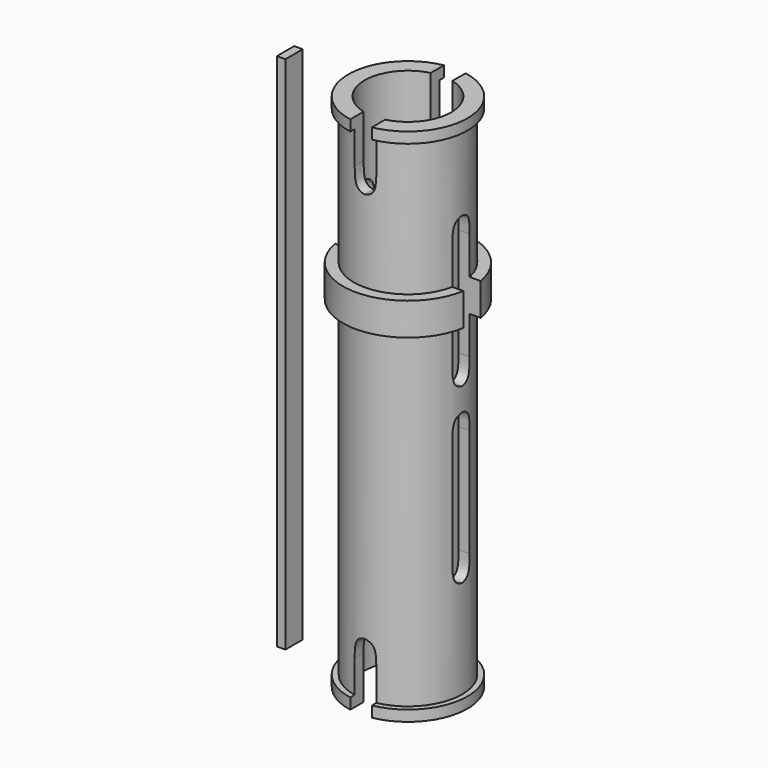
from build123d import *

# Parameters (mm, degrees)
F0_R           = 3
F1_DEPTH       = 24
F2_R           = 3
F2_R_2         = 2.5
F3_DEPTH       = 6.75
F4_R           = 2.75
F5_DEPTH       = 0.5
F6_R           = 3
F6_R_2         = 2.5
F7_DEPTH       = 6.75
F8_R           = 2.75
F9_DEPTH       = 0.5
F10_R          = 2
F11_DEPTH      = 25
F13_DEPTH      = 3
F15_DEPTH      = 3
F16_DEPTH      = 9
F17_T4_DEPTH   = 5.5129980697
F17_S5_R       = 2.5
F17_T6_DEPTH   = 4
F17_S7_R       = 2
F17_T8_DEPTH   = 4
F17_T12_DEPTH  = 5.5129980697
F17_S13_R      = 2.5
F17_T14_DEPTH  = 4
F17_S15_R      = 2
F17_T16_DEPTH  = 4
F17_T20_DEPTH  = 5.5129980697
F17_S21_R      = 2.5
F17_T22_DEPTH  = 4
F17_S23_R      = 2
F17_T24_DEPTH  = 4
F17_T28_DEPTH  = 5.5129980697
F17_S29_R      = 2.5
F17_T30_DEPTH  = 4
F17_S31_R      = 2
F17_T32_DEPTH  = 4
F17_T36_DEPTH  = 5.5129980697
F17_S37_R      = 2
F17_T38_DEPTH  = 4
F17_S39_R      = 2.5
F17_T40_DEPTH  = 4
F17_T44_DEPTH  = 5.5129980697
F17_S45_R      = 2
F17_T46_DEPTH  = 4
F17_S47_R      = 2.5
F17_T48_DEPTH  = 4
F17_T52_DEPTH  = 5.5129980697
F17_S53_R      = 2
F17_T54_DEPTH  = 4
F17_S55_R      = 2.5
F17_T56_DEPTH  = 4
F17_T60_DEPTH  = 5.5129980697
F17_S61_R      = 2
F17_T62_DEPTH  = 4
F17_S63_R      = 2.5
F17_T64_DEPTH  = 4
F19_DEPTH      = 24
F20_W          = 1
F20_H          = 7
F21_DEPTH      = 25
F22_T4_DEPTH   = 5.5129980697
F22_S5_R       = 2
F22_T6_DEPTH   = 4
F22_S7_R       = 2.5
F22_T8_DEPTH   = 4
F22_T12_DEPTH  = 5.5129980697
F22_S13_R      = 2
F22_T14_DEPTH  = 4
F22_S15_R      = 2.5
F22_T16_DEPTH  = 4
F22_T20_DEPTH  = 5.5129980697
F22_S21_R      = 2
F22_T22_DEPTH  = 4
F22_S23_R      = 2.5
F22_T24_DEPTH  = 4
F22_T28_DEPTH  = 5.5129980697
F22_S29_R      = 2
F22_T30_DEPTH  = 4
F22_S31_R      = 2.5
F22_T32_DEPTH  = 4
F22_T36_DEPTH  = 5.5129980697
F22_S37_R      = 2
F22_T38_DEPTH  = 4
F22_S39_R      = 2.5
F22_T40_DEPTH  = 4
F22_T44_DEPTH  = 5.5129980697
F22_S45_R      = 2
F22_T46_DEPTH  = 4
F22_S47_R      = 2.5
F22_T48_DEPTH  = 4
F22_T52_DEPTH  = 5.5129980697
F22_S53_R      = 2
F22_T54_DEPTH  = 4
F22_S55_R      = 2.5
F22_T56_DEPTH  = 4
F22_T60_DEPTH  = 5.5129980697
F22_S61_R      = 2
F22_T62_DEPTH  = 4
F22_S63_R      = 2.5
F22_T64_DEPTH  = 4
F22_T68_DEPTH  = 5.5129980697
F22_S69_R      = 2
F22_T70_DEPTH  = 4
F22_S71_R      = 2.5
F22_T72_DEPTH  = 4
F22_T76_DEPTH  = 5.5129980697
F22_S77_R      = 2
F22_T78_DEPTH  = 4
F22_S79_R      = 2.5
F22_T80_DEPTH  = 4
F22_T84_DEPTH  = 5.5129980697
F22_S85_R      = 2
F22_T86_DEPTH  = 4
F22_S87_R      = 2.5
F22_T88_DEPTH  = 4
F22_T92_DEPTH  = 5.5129980697
F22_S93_R      = 2.5
F22_T94_DEPTH  = 4
F22_S95_R      = 2
F22_T96_DEPTH  = 4
F22_T100_DEPTH = 5.5129980697
F22_S101_R     = 2
F22_T102_DEPTH = 4
F22_S103_R     = 2.5
F22_T104_DEPTH = 4
F22_T108_DEPTH = 5.5129980697
F22_S109_R     = 2.5
F22_T110_DEPTH = 4
F22_S111_R     = 2
F22_T112_DEPTH = 4
F22_T116_DEPTH = 5.5129980697
F22_S117_R     = 2
F22_T118_DEPTH = 4
F22_S119_R     = 2.5
F22_T120_DEPTH = 4
F22_T124_DEPTH = 5.5129980697
F22_S125_R     = 2
F22_T126_DEPTH = 4
F22_S127_R     = 2.5
F22_T128_DEPTH = 4


# Not quite as in the source:
# - a fillet or chamfer that OpenCascade refuses, or shapes differently, is made with other operations: its cross-section is extruded or revolved along the edge and cut away or added


with BuildPart() as f1:
    # F0 (on Top) → F1 (new body)
    with BuildSketch(Plane.XY):
        with Locations((-5.9236139059, -29.9984049052)):
            Circle(F0_R)
    extrude(amount=F1_DEPTH)

    # F2 (on face) → F3 (cut)
    with BuildSketch(Plane.XY.offset(24)):
        with Locations((-5.9236139059, -29.9984049052)):
            Circle(F2_R)
        with Locations((-5.9236139059, -29.9984049052)):
            Circle(F2_R_2, mode=Mode.SUBTRACT)
    extrude(amount=-F3_DEPTH, mode=Mode.SUBTRACT)

    # F4 (on face) → F5 (join)
    with BuildSketch(Plane.XY.offset(24)):
        with Locations((-5.9236139059, -29.9984049052)):
            Circle(F4_R)
    extrude(amount=-F5_DEPTH)

    # F6 (on face) → F7 (cut)
    with BuildSketch(Plane(origin=(0, 0, 0), x_dir=(1, 0, 0), z_dir=(0, 0, -1))):
        with Locations((-5.9236139059, 29.9984049052)):
            Circle(F6_R)
        with Locations((-5.9236139059, 29.9984049052)):
            Circle(F6_R_2, mode=Mode.SUBTRACT)
    extrude(amount=-F7_DEPTH, mode=Mode.SUBTRACT)

    # F8 (on face) → F9 (join)
    with BuildSketch(Plane(origin=(0, 0, 0), x_dir=(1, 0, 0), z_dir=(0, 0, -1))):
        with Locations((-5.9236139059, 29.9984049052)):
            Circle(F8_R)
    extrude(amount=-F9_DEPTH)

    # F10 (on face) → F11 (cut)
    with BuildSketch(Plane(origin=(0, 0, 0), x_dir=(1, 0, 0), z_dir=(0, 0, -1))):
        with Locations((-5.9236139059, 29.9984049052)):
            Circle(F10_R)
    extrude(amount=-F11_DEPTH, mode=Mode.SUBTRACT)

    # F12 (on face) → F13 (cut)
    with BuildSketch(Plane.XY.offset(24)):
        with BuildLine():
            ThreePointArc((-6.4236139059, -32.7025683618), (-5.9236139059, -32.7484049052), (-5.4236139059, -32.7025683618))
            Line((-5.4236139059, -32.7025683618), (-5.4236139059, -31.9348965783))
            ThreePointArc((-5.4236139059, -31.9348965783), (-5.9236139059, -31.9984049052), (-6.4236139059, -31.9348965783))
            Line((-6.4236139059, -31.9348965783), (-6.4236139059, -32.7025683618))
        make_face()
        with BuildLine():
            ThreePointArc((-5.4236139059, -27.2942414486), (-5.9236139059, -27.2484049052), (-6.4236139059, -27.2942414486))
            Line((-6.4236139059, -27.2942414486), (-6.4236139059, -28.0619132321))
            ThreePointArc((-6.4236139059, -28.0619132321), (-5.9236139059, -27.9984049052), (-5.4236139059, -28.0619132321))
            Line((-5.4236139059, -28.0619132321), (-5.4236139059, -27.2942414486))
        make_face()
    extrude(amount=-F13_DEPTH, mode=Mode.SUBTRACT)

    # F14 (on face) → F15 (cut)
    with BuildSketch(Plane(origin=(0, 0, 0), x_dir=(1, 0, 0), z_dir=(0, 0, -1))):
        Polygon((-5.4236139059, 33.0966450274), (-5.9236139059, 33.0966450274), (-6.4236139059, 33.0966450274), (-6.4236139059, 26.7786514014), (-5.4236139059, 26.7786514014), align=None)
    extrude(amount=-F15_DEPTH, mode=Mode.SUBTRACT)

    # F16 (cut): a face of the model
    f16_faces = [f1.faces().sort_by_distance(p)[0] for p in [
        (-8.8387610922, -29.9984049052, 6.75),
    ]]
    extrude(f16_faces, amount=-F16_DEPTH, mode=Mode.SUBTRACT)

    # F17: fillet of radius 1 on 8 edges, made by hand


with BuildPart() as f17_tool2:
    # F17_s3 → F17_t4 (new body)
    with BuildSketch(Plane.XZ.offset(29.4348965783)):
        with BuildLine():
            add(Edge.make_bspline(
                [(-5.4236139059, 21), (-6.4236139059, 21), (-6.4236139059, 22)],
                knots=[0, 0, 0, 1, 1, 1], degree=2, weights=[1, 1.8571428571, 1]))
            Line((-6.4236139059, 22), (-6.4236139059, 21))
            Line((-6.4236139059, 21), (-5.4236139059, 21))
        make_face()
    extrude(amount=F17_T4_DEPTH)

    # F17_s5 → F17_t6 (intersect, symmetric)
    with BuildSketch(Plane.XY.offset(21.5)):
        with Locations((-5.9236139059, -29.9984049052)):
            Circle(F17_S5_R)
    extrude(amount=F17_T6_DEPTH, both=True, mode=Mode.INTERSECT)

    # F17_s7 → F17_t8 (cut, symmetric)
    with BuildSketch(Plane.XY.offset(21.5)):
        with Locations((-5.9236139059, -29.9984049052)):
            Circle(F17_S7_R)
    extrude(amount=F17_T8_DEPTH, both=True, mode=Mode.SUBTRACT)


with BuildPart() as f1_1:
    add(f1.part)

    # F17_t1: union F17_tool2
    add(f17_tool2.part)


with BuildPart() as f17_tool10:
    # F17_s11 → F17_t12 (new body)
    with BuildSketch(Plane.XZ.offset(34.947894648)):
        with BuildLine():
            add(Edge.make_bspline(
                [(-5.4236139059, 22), (-5.4236139059, 21), (-6.4236139059, 21)],
                knots=[0, 0, 0, 1, 1, 1], degree=2, weights=[1, 1.8571428571, 1]))
            Line((-6.4236139059, 21), (-5.4236139059, 21))
            Line((-5.4236139059, 21), (-5.4236139059, 22))
        make_face()
    extrude(amount=-F17_T12_DEPTH)

    # F17_s13 → F17_t14 (intersect, symmetric)
    with BuildSketch(Plane.XY.offset(21.5)):
        with Locations((-5.9236139059, -29.9984049052)):
            Circle(F17_S13_R)
    extrude(amount=F17_T14_DEPTH, both=True, mode=Mode.INTERSECT)

    # F17_s15 → F17_t16 (cut, symmetric)
    with BuildSketch(Plane.XY.offset(21.5)):
        with Locations((-5.9236139059, -29.9984049052)):
            Circle(F17_S15_R)
    extrude(amount=F17_T16_DEPTH, both=True, mode=Mode.SUBTRACT)


with BuildPart() as f1_2:
    add(f1_1.part)

    # F17_t9: union F17_tool10
    add(f17_tool10.part)


with BuildPart() as f17_tool18:
    # F17_s19 → F17_t20 (new body)
    with BuildSketch(Plane.XZ.offset(30.5619132321)):
        with BuildLine():
            add(Edge.make_bspline(
                [(-6.4236139059, 21), (-5.4236139059, 21), (-5.4236139059, 22)],
                knots=[0, 0, 0, 1, 1, 1], degree=2, weights=[1, 1.8571428571, 1]))
            Line((-5.4236139059, 22), (-5.4236139059, 21))
            Line((-5.4236139059, 21), (-6.4236139059, 21))
        make_face()
    extrude(amount=-F17_T20_DEPTH)

    # F17_s21 → F17_t22 (intersect, symmetric)
    with BuildSketch(Plane.XY.offset(21.5)):
        with Locations((-5.9236139059, -29.9984049052)):
            Circle(F17_S21_R)
    extrude(amount=F17_T22_DEPTH, both=True, mode=Mode.INTERSECT)

    # F17_s23 → F17_t24 (cut, symmetric)
    with BuildSketch(Plane.XY.offset(21.5)):
        with Locations((-5.9236139059, -29.9984049052)):
            Circle(F17_S23_R)
    extrude(amount=F17_T24_DEPTH, both=True, mode=Mode.SUBTRACT)


with BuildPart() as f1_3:
    add(f1_2.part)

    # F17_t17: union F17_tool18
    add(f17_tool18.part)


with BuildPart() as f17_tool26:
    # F17_s27 → F17_t28 (new body)
    with BuildSketch(Plane.XZ.offset(25.0489151624)):
        with BuildLine():
            add(Edge.make_bspline(
                [(-6.4236139059, 22), (-6.4236139059, 21), (-5.4236139059, 21)],
                knots=[0, 0, 0, 1, 1, 1], degree=2, weights=[1, 1.8571428571, 1]))
            Line((-5.4236139059, 21), (-6.4236139059, 21))
            Line((-6.4236139059, 21), (-6.4236139059, 22))
        make_face()
    extrude(amount=F17_T28_DEPTH)

    # F17_s29 → F17_t30 (intersect, symmetric)
    with BuildSketch(Plane.XY.offset(21.5)):
        with Locations((-5.9236139059, -29.9984049052)):
            Circle(F17_S29_R)
    extrude(amount=F17_T30_DEPTH, both=True, mode=Mode.INTERSECT)

    # F17_s31 → F17_t32 (cut, symmetric)
    with BuildSketch(Plane.XY.offset(21.5)):
        with Locations((-5.9236139059, -29.9984049052)):
            Circle(F17_S31_R)
    extrude(amount=F17_T32_DEPTH, both=True, mode=Mode.SUBTRACT)


with BuildPart() as f1_4:
    add(f1_3.part)

    # F17_t25: union F17_tool26
    add(f17_tool26.part)


with BuildPart() as f17_tool34:
    # F17_s35 → F17_t36 (new body)
    with BuildSketch(Plane.XZ.offset(25.0489151624)):
        with BuildLine():
            add(Edge.make_bspline(
                [(-5.4236139059, 2), (-5.4236139059, 3), (-6.4236139059, 3)],
                knots=[0, 0, 0, 1, 1, 1], degree=2, weights=[1, 1.8571428571, 1]))
            Line((-6.4236139059, 3), (-5.4236139059, 3))
            Line((-5.4236139059, 3), (-5.4236139059, 2))
        make_face()
    extrude(amount=F17_T36_DEPTH)

    # F17_s37 → F17_t38 (cut, symmetric)
    with BuildSketch(Plane.XY.offset(2.5)):
        with Locations((-5.9236139059, -29.9984049052)):
            Circle(F17_S37_R)
    extrude(amount=F17_T38_DEPTH, both=True, mode=Mode.SUBTRACT)

    # F17_s39 → F17_t40 (intersect, symmetric)
    with BuildSketch(Plane.XY.offset(2.5)):
        with Locations((-5.9236139059, -29.9984049052)):
            Circle(F17_S39_R)
    extrude(amount=F17_T40_DEPTH, both=True, mode=Mode.INTERSECT)


with BuildPart() as f1_5:
    add(f1_4.part)

    # F17_t33: union F17_tool34
    add(f17_tool34.part)


with BuildPart() as f17_tool42:
    # F17_s43 → F17_t44 (new body)
    with BuildSketch(Plane.XZ.offset(29.4348965783)):
        with BuildLine():
            add(Edge.make_bspline(
                [(-6.4236139059, 3), (-5.4236139059, 3), (-5.4236139059, 2)],
                knots=[0, 0, 0, 1, 1, 1], degree=2, weights=[1, 1.8571428571, 1]))
            Line((-5.4236139059, 2), (-5.4236139059, 3))
            Line((-5.4236139059, 3), (-6.4236139059, 3))
        make_face()
    extrude(amount=F17_T44_DEPTH)

    # F17_s45 → F17_t46 (cut, symmetric)
    with BuildSketch(Plane.XY.offset(2.5)):
        with Locations((-5.9236139059, -29.9984049052)):
            Circle(F17_S45_R)
    extrude(amount=F17_T46_DEPTH, both=True, mode=Mode.SUBTRACT)

    # F17_s47 → F17_t48 (intersect, symmetric)
    with BuildSketch(Plane.XY.offset(2.5)):
        with Locations((-5.9236139059, -29.9984049052)):
            Circle(F17_S47_R)
    extrude(amount=F17_T48_DEPTH, both=True, mode=Mode.INTERSECT)


with BuildPart() as f1_6:
    add(f1_5.part)

    # F17_t41: union F17_tool42
    add(f17_tool42.part)


with BuildPart() as f17_tool50:
    # F17_s51 → F17_t52 (new body)
    with BuildSketch(Plane.XZ.offset(30.5619132321)):
        with BuildLine():
            add(Edge.make_bspline(
                [(-5.4236139059, 3), (-6.4236139059, 3), (-6.4236139059, 2)],
                knots=[0, 0, 0, 1, 1, 1], degree=2, weights=[1, 1.8571428571, 1]))
            Line((-6.4236139059, 2), (-6.4236139059, 3))
            Line((-6.4236139059, 3), (-5.4236139059, 3))
        make_face()
    extrude(amount=-F17_T52_DEPTH)

    # F17_s53 → F17_t54 (cut, symmetric)
    with BuildSketch(Plane.XY.offset(2.5)):
        with Locations((-5.9236139059, -29.9984049052)):
            Circle(F17_S53_R)
    extrude(amount=F17_T54_DEPTH, both=True, mode=Mode.SUBTRACT)

    # F17_s55 → F17_t56 (intersect, symmetric)
    with BuildSketch(Plane.XY.offset(2.5)):
        with Locations((-5.9236139059, -29.9984049052)):
            Circle(F17_S55_R)
    extrude(amount=F17_T56_DEPTH, both=True, mode=Mode.INTERSECT)


with BuildPart() as f1_7:
    add(f1_6.part)

    # F17_t49: union F17_tool50
    add(f17_tool50.part)


with BuildPart() as f17_tool58:
    # F17_s59 → F17_t60 (new body)
    with BuildSketch(Plane.XZ.offset(34.947894648)):
        with BuildLine():
            add(Edge.make_bspline(
                [(-6.4236139059, 2), (-6.4236139059, 3), (-5.4236139059, 3)],
                knots=[0, 0, 0, 1, 1, 1], degree=2, weights=[1, 1.8571428571, 1]))
            Line((-5.4236139059, 3), (-6.4236139059, 3))
            Line((-6.4236139059, 3), (-6.4236139059, 2))
        make_face()
    extrude(amount=-F17_T60_DEPTH)

    # F17_s61 → F17_t62 (cut, symmetric)
    with BuildSketch(Plane.XY.offset(2.5)):
        with Locations((-5.9236139059, -29.9984049052)):
            Circle(F17_S61_R)
    extrude(amount=F17_T62_DEPTH, both=True, mode=Mode.SUBTRACT)

    # F17_s63 → F17_t64 (intersect, symmetric)
    with BuildSketch(Plane.XY.offset(2.5)):
        with Locations((-5.9236139059, -29.9984049052)):
            Circle(F17_S63_R)
    extrude(amount=F17_T64_DEPTH, both=True, mode=Mode.INTERSECT)


with BuildPart() as f1_8:
    add(f1_7.part)

    # F17_t57: union F17_tool58
    add(f17_tool58.part)

    # F20 (on face) → F21 (cut)
    with BuildSketch(Plane(origin=(-11.5753058344, 0, 0), x_dir=(0, -1, 0), z_dir=(-1, 0, 0))):
        Polygon((30.4984049052, 20), (29.4984049052, 20), (29.4984049052, 16.5), (29.4984049052, 13), (30.4984049052, 13), align=None)
        with Locations((29.9984049052, 8.5)):
            Rectangle(F20_W, F20_H)
    extrude(amount=-F21_DEPTH, mode=Mode.SUBTRACT)

    # F22: fillet of radius 1 on 16 edges, made by hand


with BuildPart() as f19:
    # F18 (on face) → F19 (new body)
    with BuildSketch(Plane(origin=(0, 0, 0), x_dir=(1, 0, 0), z_dir=(0, 0, -1))):
        Polygon((-11.5753058344, 30.4984049052), (-11.5753058344, 29.9984049052), (-11.5753058344, 29.4984049052), (-11.1821657047, 29.4984049052), (-11.1821657047, 30.4984049052), align=None)
    extrude(amount=-F19_DEPTH)


with BuildPart() as f22_tool2:
    # F22_s3 → F22_t4 (new body)
    with BuildSketch(Plane.YZ.offset(-6.4871222328)):
        with BuildLine():
            add(Edge.make_bspline(
                [(-29.4984049052, 5), (-30.4984049052, 5), (-30.4984049052, 6)],
                knots=[0, 0, 0, 1, 1, 1], degree=2, weights=[1, 1.8571428571, 1]))
            Line((-30.4984049052, 6), (-30.4984049052, 5))
            Line((-30.4984049052, 5), (-29.4984049052, 5))
        make_face()
    extrude(amount=F22_T4_DEPTH)

    # F22_s5 → F22_t6 (cut, symmetric)
    with BuildSketch(Plane.XY.offset(5.5)):
        with Locations((-5.9236139059, -29.9984049052)):
            Circle(F22_S5_R)
    extrude(amount=F22_T6_DEPTH, both=True, mode=Mode.SUBTRACT)

    # F22_s7 → F22_t8 (intersect, symmetric)
    with BuildSketch(Plane.XY.offset(5.5)):
        with Locations((-5.9236139059, -29.9984049052)):
            Circle(F22_S7_R)
    extrude(amount=F22_T8_DEPTH, both=True, mode=Mode.INTERSECT)


with BuildPart() as f1_9:
    add(f1_8.part)

    # F22_t1: union F22_tool2
    add(f22_tool2.part)


with BuildPart() as f22_tool10:
    # F22_s11 → F22_t12 (new body)
    with BuildSketch(Plane.YZ.offset(-10.8731036487)):
        with BuildLine():
            add(Edge.make_bspline(
                [(-29.4984049052, 5), (-30.4984049052, 5), (-30.4984049052, 6)],
                knots=[0, 0, 0, 1, 1, 1], degree=2, weights=[1, 1.8571428571, 1]))
            Line((-30.4984049052, 6), (-30.4984049052, 5))
            Line((-30.4984049052, 5), (-29.4984049052, 5))
        make_face()
    extrude(amount=F22_T12_DEPTH)

    # F22_s13 → F22_t14 (cut, symmetric)
    with BuildSketch(Plane.XY.offset(5.5)):
        with Locations((-5.9236139059, -29.9984049052)):
            Circle(F22_S13_R)
    extrude(amount=F22_T14_DEPTH, both=True, mode=Mode.SUBTRACT)

    # F22_s15 → F22_t16 (intersect, symmetric)
    with BuildSketch(Plane.XY.offset(5.5)):
        with Locations((-5.9236139059, -29.9984049052)):
            Circle(F22_S15_R)
    extrude(amount=F22_T16_DEPTH, both=True, mode=Mode.INTERSECT)


with BuildPart() as f1_10:
    add(f1_9.part)

    # F22_t9: union F22_tool10
    add(f22_tool10.part)


with BuildPart() as f22_tool18:
    # F22_s19 → F22_t20 (new body)
    with BuildSketch(Plane.YZ.offset(-6.4871222328)):
        with BuildLine():
            add(Edge.make_bspline(
                [(-30.4984049052, 5), (-29.4984049052, 5), (-29.4984049052, 6)],
                knots=[0, 0, 0, 1, 1, 1], degree=2, weights=[1, 1.8571428571, 1]))
            Line((-29.4984049052, 6), (-29.4984049052, 5))
            Line((-29.4984049052, 5), (-30.4984049052, 5))
        make_face()
    extrude(amount=F22_T20_DEPTH)

    # F22_s21 → F22_t22 (cut, symmetric)
    with BuildSketch(Plane.XY.offset(5.5)):
        with Locations((-5.9236139059, -29.9984049052)):
            Circle(F22_S21_R)
    extrude(amount=F22_T22_DEPTH, both=True, mode=Mode.SUBTRACT)

    # F22_s23 → F22_t24 (intersect, symmetric)
    with BuildSketch(Plane.XY.offset(5.5)):
        with Locations((-5.9236139059, -29.9984049052)):
            Circle(F22_S23_R)
    extrude(amount=F22_T24_DEPTH, both=True, mode=Mode.INTERSECT)


with BuildPart() as f1_11:
    add(f1_10.part)

    # F22_t17: union F22_tool18
    add(f22_tool18.part)


with BuildPart() as f22_tool26:
    # F22_s27 → F22_t28 (new body)
    with BuildSketch(Plane.YZ.offset(-10.8731036487)):
        with BuildLine():
            add(Edge.make_bspline(
                [(-29.4984049052, 6), (-29.4984049052, 5), (-30.4984049052, 5)],
                knots=[0, 0, 0, 1, 1, 1], degree=2, weights=[1, 1.8571428571, 1]))
            Line((-30.4984049052, 5), (-29.4984049052, 5))
            Line((-29.4984049052, 5), (-29.4984049052, 6))
        make_face()
    extrude(amount=F22_T28_DEPTH)

    # F22_s29 → F22_t30 (cut, symmetric)
    with BuildSketch(Plane.XY.offset(5.5)):
        with Locations((-5.9236139059, -29.9984049052)):
            Circle(F22_S29_R)
    extrude(amount=F22_T30_DEPTH, both=True, mode=Mode.SUBTRACT)

    # F22_s31 → F22_t32 (intersect, symmetric)
    with BuildSketch(Plane.XY.offset(5.5)):
        with Locations((-5.9236139059, -29.9984049052)):
            Circle(F22_S31_R)
    extrude(amount=F22_T32_DEPTH, both=True, mode=Mode.INTERSECT)


with BuildPart() as f1_12:
    add(f1_11.part)

    # F22_t25: union F22_tool26
    add(f22_tool26.part)


with BuildPart() as f22_tool34:
    # F22_s35 → F22_t36 (new body)
    with BuildSketch(Plane.YZ.offset(-6.4871222328)):
        with BuildLine():
            add(Edge.make_bspline(
                [(-29.4984049052, 12), (-30.4984049052, 12), (-30.4984049052, 11)],
                knots=[0, 0, 0, 1, 1, 1], degree=2, weights=[1, 1.8571428571, 1]))
            Line((-30.4984049052, 11), (-30.4984049052, 12))
            Line((-30.4984049052, 12), (-29.4984049052, 12))
        make_face()
    extrude(amount=F22_T36_DEPTH)

    # F22_s37 → F22_t38 (cut, symmetric)
    with BuildSketch(Plane.XY.offset(11.5)):
        with Locations((-5.9236139059, -29.9984049052)):
            Circle(F22_S37_R)
    extrude(amount=F22_T38_DEPTH, both=True, mode=Mode.SUBTRACT)

    # F22_s39 → F22_t40 (intersect, symmetric)
    with BuildSketch(Plane.XY.offset(11.5)):
        with Locations((-5.9236139059, -29.9984049052)):
            Circle(F22_S39_R)
    extrude(amount=F22_T40_DEPTH, both=True, mode=Mode.INTERSECT)


with BuildPart() as f1_13:
    add(f1_12.part)

    # F22_t33: union F22_tool34
    add(f22_tool34.part)


with BuildPart() as f22_tool42:
    # F22_s43 → F22_t44 (new body)
    with BuildSketch(Plane.YZ.offset(-10.8731036487)):
        with BuildLine():
            add(Edge.make_bspline(
                [(-29.4984049052, 12), (-30.4984049052, 12), (-30.4984049052, 11)],
                knots=[0, 0, 0, 1, 1, 1], degree=2, weights=[1, 1.8571428571, 1]))
            Line((-30.4984049052, 11), (-30.4984049052, 12))
            Line((-30.4984049052, 12), (-29.4984049052, 12))
        make_face()
    extrude(amount=F22_T44_DEPTH)

    # F22_s45 → F22_t46 (cut, symmetric)
    with BuildSketch(Plane.XY.offset(11.5)):
        with Locations((-5.9236139059, -29.9984049052)):
            Circle(F22_S45_R)
    extrude(amount=F22_T46_DEPTH, both=True, mode=Mode.SUBTRACT)

    # F22_s47 → F22_t48 (intersect, symmetric)
    with BuildSketch(Plane.XY.offset(11.5)):
        with Locations((-5.9236139059, -29.9984049052)):
            Circle(F22_S47_R)
    extrude(amount=F22_T48_DEPTH, both=True, mode=Mode.INTERSECT)


with BuildPart() as f1_14:
    add(f1_13.part)

    # F22_t41: union F22_tool42
    add(f22_tool42.part)


with BuildPart() as f22_tool50:
    # F22_s51 → F22_t52 (new body)
    with BuildSketch(Plane.YZ.offset(-6.4871222328)):
        with BuildLine():
            add(Edge.make_bspline(
                [(-29.4984049052, 11), (-29.4984049052, 12), (-30.4984049052, 12)],
                knots=[0, 0, 0, 1, 1, 1], degree=2, weights=[1, 1.8571428571, 1]))
            Line((-30.4984049052, 12), (-29.4984049052, 12))
            Line((-29.4984049052, 12), (-29.4984049052, 11))
        make_face()
    extrude(amount=F22_T52_DEPTH)

    # F22_s53 → F22_t54 (cut, symmetric)
    with BuildSketch(Plane.XY.offset(11.5)):
        with Locations((-5.9236139059, -29.9984049052)):
            Circle(F22_S53_R)
    extrude(amount=F22_T54_DEPTH, both=True, mode=Mode.SUBTRACT)

    # F22_s55 → F22_t56 (intersect, symmetric)
    with BuildSketch(Plane.XY.offset(11.5)):
        with Locations((-5.9236139059, -29.9984049052)):
            Circle(F22_S55_R)
    extrude(amount=F22_T56_DEPTH, both=True, mode=Mode.INTERSECT)


with BuildPart() as f1_15:
    add(f1_14.part)

    # F22_t49: union F22_tool50
    add(f22_tool50.part)


with BuildPart() as f22_tool58:
    # F22_s59 → F22_t60 (new body)
    with BuildSketch(Plane.YZ.offset(-10.8731036487)):
        with BuildLine():
            add(Edge.make_bspline(
                [(-30.4984049052, 12), (-29.4984049052, 12), (-29.4984049052, 11)],
                knots=[0, 0, 0, 1, 1, 1], degree=2, weights=[1, 1.8571428571, 1]))
            Line((-29.4984049052, 11), (-29.4984049052, 12))
            Line((-29.4984049052, 12), (-30.4984049052, 12))
        make_face()
    extrude(amount=F22_T60_DEPTH)

    # F22_s61 → F22_t62 (cut, symmetric)
    with BuildSketch(Plane.XY.offset(11.5)):
        with Locations((-5.9236139059, -29.9984049052)):
            Circle(F22_S61_R)
    extrude(amount=F22_T62_DEPTH, both=True, mode=Mode.SUBTRACT)

    # F22_s63 → F22_t64 (intersect, symmetric)
    with BuildSketch(Plane.XY.offset(11.5)):
        with Locations((-5.9236139059, -29.9984049052)):
            Circle(F22_S63_R)
    extrude(amount=F22_T64_DEPTH, both=True, mode=Mode.INTERSECT)


with BuildPart() as f1_16:
    add(f1_15.part)

    # F22_t57: union F22_tool58
    add(f22_tool58.part)


with BuildPart() as f22_tool66:
    # F22_s67 → F22_t68 (new body)
    with BuildSketch(Plane.YZ.offset(-6.4871222328)):
        with BuildLine():
            add(Edge.make_bspline(
                [(-30.4984049052, 13), (-29.4984049052, 13), (-29.4984049052, 14)],
                knots=[0, 0, 0, 1, 1, 1], degree=2, weights=[1, 1.8571428571, 1]))
            Line((-29.4984049052, 14), (-29.4984049052, 13))
            Line((-29.4984049052, 13), (-30.4984049052, 13))
        make_face()
    extrude(amount=F22_T68_DEPTH)

    # F22_s69 → F22_t70 (cut, symmetric)
    with BuildSketch(Plane.XY.offset(13.5)):
        with Locations((-5.9236139059, -29.9984049052)):
            Circle(F22_S69_R)
    extrude(amount=F22_T70_DEPTH, both=True, mode=Mode.SUBTRACT)

    # F22_s71 → F22_t72 (intersect, symmetric)
    with BuildSketch(Plane.XY.offset(13.5)):
        with Locations((-5.9236139059, -29.9984049052)):
            Circle(F22_S71_R)
    extrude(amount=F22_T72_DEPTH, both=True, mode=Mode.INTERSECT)


with BuildPart() as f1_17:
    add(f1_16.part)

    # F22_t65: union F22_tool66
    add(f22_tool66.part)


with BuildPart() as f22_tool74:
    # F22_s75 → F22_t76 (new body)
    with BuildSketch(Plane.YZ.offset(-10.8731036487)):
        with BuildLine():
            add(Edge.make_bspline(
                [(-30.4984049052, 13), (-29.4984049052, 13), (-29.4984049052, 14)],
                knots=[0, 0, 0, 1, 1, 1], degree=2, weights=[1, 1.8571428571, 1]))
            Line((-29.4984049052, 14), (-29.4984049052, 13))
            Line((-29.4984049052, 13), (-30.4984049052, 13))
        make_face()
    extrude(amount=F22_T76_DEPTH)

    # F22_s77 → F22_t78 (cut, symmetric)
    with BuildSketch(Plane.XY.offset(13.5)):
        with Locations((-5.9236139059, -29.9984049052)):
            Circle(F22_S77_R)
    extrude(amount=F22_T78_DEPTH, both=True, mode=Mode.SUBTRACT)

    # F22_s79 → F22_t80 (intersect, symmetric)
    with BuildSketch(Plane.XY.offset(13.5)):
        with Locations((-5.9236139059, -29.9984049052)):
            Circle(F22_S79_R)
    extrude(amount=F22_T80_DEPTH, both=True, mode=Mode.INTERSECT)


with BuildPart() as f1_18:
    add(f1_17.part)

    # F22_t73: union F22_tool74
    add(f22_tool74.part)


with BuildPart() as f22_tool82:
    # F22_s83 → F22_t84 (new body)
    with BuildSketch(Plane.YZ.offset(-6.4871222328)):
        with BuildLine():
            add(Edge.make_bspline(
                [(-30.4984049052, 14), (-30.4984049052, 13), (-29.4984049052, 13)],
                knots=[0, 0, 0, 1, 1, 1], degree=2, weights=[1, 1.8571428571, 1]))
            Line((-29.4984049052, 13), (-30.4984049052, 13))
            Line((-30.4984049052, 13), (-30.4984049052, 14))
        make_face()
    extrude(amount=F22_T84_DEPTH)

    # F22_s85 → F22_t86 (cut, symmetric)
    with BuildSketch(Plane.XY.offset(13.5)):
        with Locations((-5.9236139059, -29.9984049052)):
            Circle(F22_S85_R)
    extrude(amount=F22_T86_DEPTH, both=True, mode=Mode.SUBTRACT)

    # F22_s87 → F22_t88 (intersect, symmetric)
    with BuildSketch(Plane.XY.offset(13.5)):
        with Locations((-5.9236139059, -29.9984049052)):
            Circle(F22_S87_R)
    extrude(amount=F22_T88_DEPTH, both=True, mode=Mode.INTERSECT)


with BuildPart() as f1_19:
    add(f1_18.part)

    # F22_t81: union F22_tool82
    add(f22_tool82.part)


with BuildPart() as f22_tool90:
    # F22_s91 → F22_t92 (new body)
    with BuildSketch(Plane.YZ.offset(-10.8731036487)):
        with BuildLine():
            add(Edge.make_bspline(
                [(-30.4984049052, 14), (-30.4984049052, 13), (-29.4984049052, 13)],
                knots=[0, 0, 0, 1, 1, 1], degree=2, weights=[1, 1.8571428571, 1]))
            Line((-29.4984049052, 13), (-30.4984049052, 13))
            Line((-30.4984049052, 13), (-30.4984049052, 14))
        make_face()
    extrude(amount=F22_T92_DEPTH)

    # F22_s93 → F22_t94 (intersect, symmetric)
    with BuildSketch(Plane.XY.offset(13.5)):
        with Locations((-5.9236139059, -29.9984049052)):
            Circle(F22_S93_R)
    extrude(amount=F22_T94_DEPTH, both=True, mode=Mode.INTERSECT)

    # F22_s95 → F22_t96 (cut, symmetric)
    with BuildSketch(Plane.XY.offset(13.5)):
        with Locations((-5.9236139059, -29.9984049052)):
            Circle(F22_S95_R)
    extrude(amount=F22_T96_DEPTH, both=True, mode=Mode.SUBTRACT)


with BuildPart() as f1_20:
    add(f1_19.part)

    # F22_t89: union F22_tool90
    add(f22_tool90.part)


with BuildPart() as f22_tool98:
    # F22_s99 → F22_t100 (new body)
    with BuildSketch(Plane.YZ.offset(-6.4871222328)):
        with BuildLine():
            add(Edge.make_bspline(
                [(-30.4984049052, 19), (-30.4984049052, 20), (-29.4984049052, 20)],
                knots=[0, 0, 0, 1, 1, 1], degree=2, weights=[1, 1.8571428571, 1]))
            Line((-29.4984049052, 20), (-30.4984049052, 20))
            Line((-30.4984049052, 20), (-30.4984049052, 19))
        make_face()
    extrude(amount=F22_T100_DEPTH)

    # F22_s101 → F22_t102 (cut, symmetric)
    with BuildSketch(Plane.XY.offset(19.5)):
        with Locations((-5.9236139059, -29.9984049052)):
            Circle(F22_S101_R)
    extrude(amount=F22_T102_DEPTH, both=True, mode=Mode.SUBTRACT)

    # F22_s103 → F22_t104 (intersect, symmetric)
    with BuildSketch(Plane.XY.offset(19.5)):
        with Locations((-5.9236139059, -29.9984049052)):
            Circle(F22_S103_R)
    extrude(amount=F22_T104_DEPTH, both=True, mode=Mode.INTERSECT)


with BuildPart() as f1_21:
    add(f1_20.part)

    # F22_t97: union F22_tool98
    add(f22_tool98.part)


with BuildPart() as f22_tool106:
    # F22_s107 → F22_t108 (new body)
    with BuildSketch(Plane.YZ.offset(-10.8731036487)):
        with BuildLine():
            add(Edge.make_bspline(
                [(-30.4984049052, 19), (-30.4984049052, 20), (-29.4984049052, 20)],
                knots=[0, 0, 0, 1, 1, 1], degree=2, weights=[1, 1.8571428571, 1]))
            Line((-29.4984049052, 20), (-30.4984049052, 20))
            Line((-30.4984049052, 20), (-30.4984049052, 19))
        make_face()
    extrude(amount=F22_T108_DEPTH)

    # F22_s109 → F22_t110 (intersect, symmetric)
    with BuildSketch(Plane.XY.offset(19.5)):
        with Locations((-5.9236139059, -29.9984049052)):
            Circle(F22_S109_R)
    extrude(amount=F22_T110_DEPTH, both=True, mode=Mode.INTERSECT)

    # F22_s111 → F22_t112 (cut, symmetric)
    with BuildSketch(Plane.XY.offset(19.5)):
        with Locations((-5.9236139059, -29.9984049052)):
            Circle(F22_S111_R)
    extrude(amount=F22_T112_DEPTH, both=True, mode=Mode.SUBTRACT)


with BuildPart() as f1_22:
    add(f1_21.part)

    # F22_t105: union F22_tool106
    add(f22_tool106.part)


with BuildPart() as f22_tool114:
    # F22_s115 → F22_t116 (new body)
    with BuildSketch(Plane.YZ.offset(-6.4871222328)):
        with BuildLine():
            add(Edge.make_bspline(
                [(-30.4984049052, 20), (-29.4984049052, 20), (-29.4984049052, 19)],
                knots=[0, 0, 0, 1, 1, 1], degree=2, weights=[1, 1.8571428571, 1]))
            Line((-29.4984049052, 19), (-29.4984049052, 20))
            Line((-29.4984049052, 20), (-30.4984049052, 20))
        make_face()
    extrude(amount=F22_T116_DEPTH)

    # F22_s117 → F22_t118 (cut, symmetric)
    with BuildSketch(Plane.XY.offset(19.5)):
        with Locations((-5.9236139059, -29.9984049052)):
            Circle(F22_S117_R)
    extrude(amount=F22_T118_DEPTH, both=True, mode=Mode.SUBTRACT)

    # F22_s119 → F22_t120 (intersect, symmetric)
    with BuildSketch(Plane.XY.offset(19.5)):
        with Locations((-5.9236139059, -29.9984049052)):
            Circle(F22_S119_R)
    extrude(amount=F22_T120_DEPTH, both=True, mode=Mode.INTERSECT)


with BuildPart() as f1_23:
    add(f1_22.part)

    # F22_t113: union F22_tool114
    add(f22_tool114.part)


with BuildPart() as f22_tool122:
    # F22_s123 → F22_t124 (new body)
    with BuildSketch(Plane.YZ.offset(-10.8731036487)):
        with BuildLine():
            add(Edge.make_bspline(
                [(-30.4984049052, 20), (-29.4984049052, 20), (-29.4984049052, 19)],
                knots=[0, 0, 0, 1, 1, 1], degree=2, weights=[1, 1.8571428571, 1]))
            Line((-29.4984049052, 19), (-29.4984049052, 20))
            Line((-29.4984049052, 20), (-30.4984049052, 20))
        make_face()
    extrude(amount=F22_T124_DEPTH)

    # F22_s125 → F22_t126 (cut, symmetric)
    with BuildSketch(Plane.XY.offset(19.5)):
        with Locations((-5.9236139059, -29.9984049052)):
            Circle(F22_S125_R)
    extrude(amount=F22_T126_DEPTH, both=True, mode=Mode.SUBTRACT)

    # F22_s127 → F22_t128 (intersect, symmetric)
    with BuildSketch(Plane.XY.offset(19.5)):
        with Locations((-5.9236139059, -29.9984049052)):
            Circle(F22_S127_R)
    extrude(amount=F22_T128_DEPTH, both=True, mode=Mode.INTERSECT)


with BuildPart() as f1_24:
    add(f1_23.part)

    # F22_t121: union F22_tool122
    add(f22_tool122.part)


solid = Compound([f19.part, f1_24.part])
